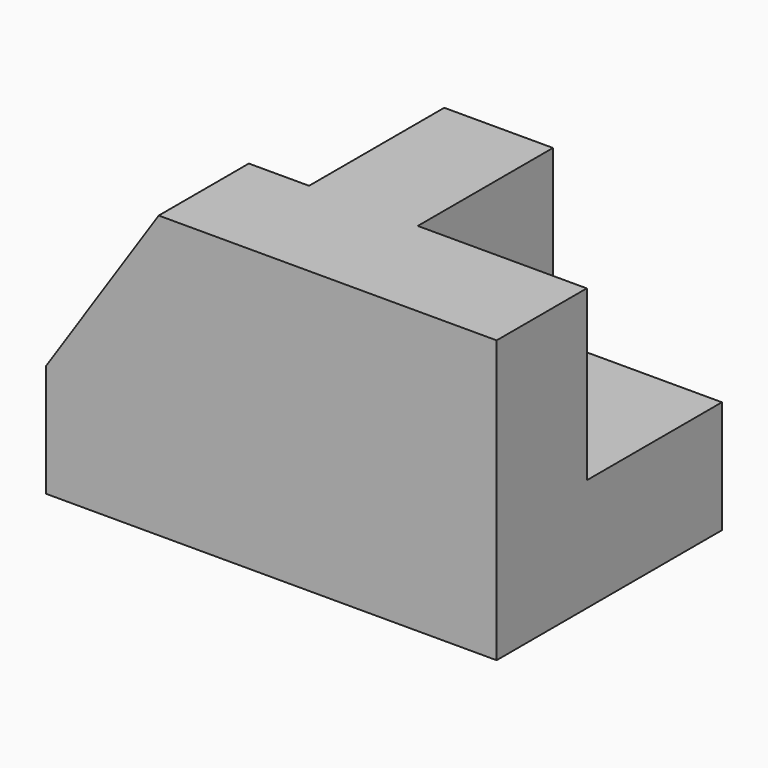
from build123d import *

# Parameters (mm, degrees)
F1_DEPTH = 31.75
F2_W     = 19.05
F2_H     = 19.05
F3_DEPTH = 19.05
F5_DEPTH = 19.05
F7_DEPTH = 19.05


# Not quite as in the source:
# - a length typed as a fraction of an inch, garbled in the dataset ("3 / 203.2 mm" for 3/8 in), is restored


with BuildPart() as f1:
    # F0 (on Front) → F1 (new body)
    with BuildSketch(Plane.XZ):
        Polygon((-50.8, 0), (0, 0), (0, 31.75), (-38.1, 31.75), (-50.8, 12.7), align=None)
    extrude(amount=F1_DEPTH)

    # F2 (on Front) → F3 (cut)
    with BuildSketch(Plane.XZ):
        with Locations((-9.525, 22.225)):
            Rectangle(F2_W, F2_H)
    extrude(amount=F3_DEPTH, mode=Mode.SUBTRACT)

    # F4 (on Front) → F5 (cut)
    with BuildSketch(Plane.XZ):
        Polygon((-31.6195416782, 13.0910674021), (-31.3020864666, 32.1384221315), (-37.6520864666, 32.1384221315), (-50.6695416782, 13.0910674021), align=None)
    extrude(amount=F5_DEPTH, mode=Mode.SUBTRACT)

    # F6 (on Front) → F7 (cut)
    with BuildSketch(Plane.XZ):
        Polygon((-34.3563221395, 12.8449322656), (-34.3563221395, 35.7176738393), (-68.0936202407, 12.8449322656), align=None)
    extrude(amount=F7_DEPTH, mode=Mode.SUBTRACT)


solid = f1.part
